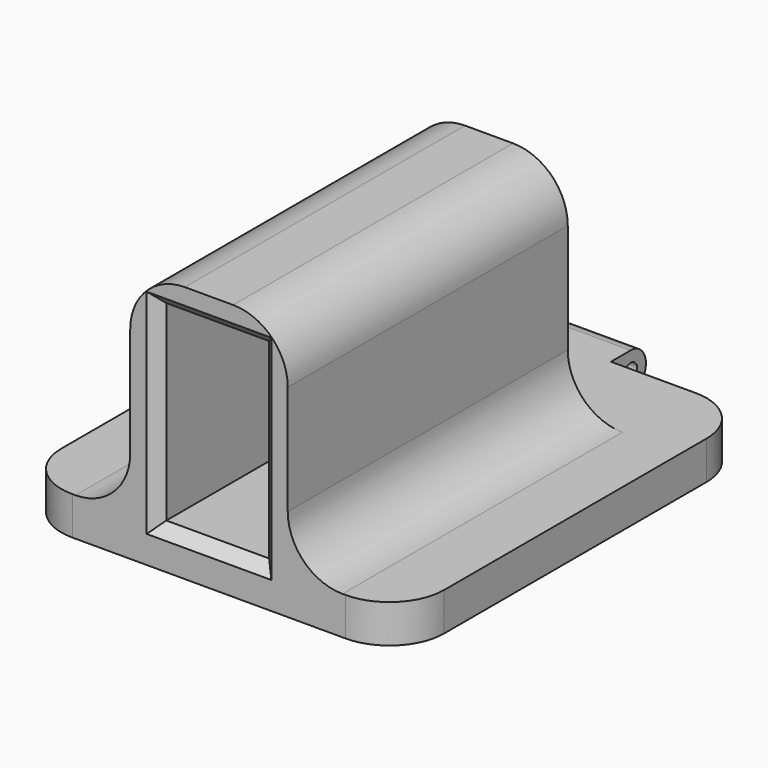
from build123d import *

# Parameters (mm, degrees)
F0_W     = 9.5
F0_H     = 4
F1_DEPTH = 3.5
F2_R     = 1.74999
F3_R     = 0.75
F4_DEPTH = 10
F5_W     = 2.5
F5_H     = 32
F6_DEPTH = 17.5
F7_W     = 14.4
F7_H     = 32
F8_DEPTH = 2.5
F9_R     = 5
F10_SIZE = 1


# Not quite as in the source:
# - a fillet or chamfer is up to 0.001 mm smaller than in the source, because OpenCascade refuses the exact size


with BuildPart() as f1:
    # F0 (on Top) → F1 (new body)
    with BuildSketch(Plane.XY):
        Polygon((0, 40), (0, 0), (35, 0), (35, 40), (22.25, 40), (12.75, 40), align=None)
        with Locations((17.5, 42)):
            Rectangle(F0_W, F0_H)
    extrude(amount=F1_DEPTH)

    # F2 (radius 1.75 in the source; OpenCascade refuses exactly that, so slightly less here)
    f2_edges = [f1.edges().sort_by_distance(p)[0] for p in [
        (17.5, 44, 3.5),
        (17.5, 44, 0),
    ]]
    fillet(f2_edges, radius=F2_R)

    # F3 (on face) → F4 (cut)
    with BuildSketch(Plane.YZ.offset(22.25)):
        with Locations((42.25, 1.75)):
            Circle(F3_R)
    extrude(amount=-F4_DEPTH, mode=Mode.SUBTRACT)

    # F5 (on face) → F6 (join)
    with BuildSketch(Plane.XY.offset(3.5)):
        with Locations((11.55, 16)):
            Rectangle(F5_W, F5_H)
        with Locations((23.45, 16)):
            Rectangle(F5_W, F5_H)
    extrude(amount=F6_DEPTH)

    # F7 (on face) → F8 (join)
    with BuildSketch(Plane.XY.offset(21)):
        with Locations((17.5, 16)):
            Rectangle(F7_W, F7_H)
    extrude(amount=F8_DEPTH)

    # F9
    f9_edges = [f1.edges().sort_by_distance(p)[0] for p in [
        (24.7, 16, 23.5),
        (10.3, 16, 23.5),
        (24.7, 16, 3.5),
        (10.3, 16, 3.5),
        (35, 40, 1.75),
        (0, 40, 1.75),
        (0, 0, 1.75),
        (35, 0, 1.75),
    ]]
    fillet(f9_edges, radius=F9_R)

    # F10
    f10_edges = [f1.edges().sort_by_distance(p)[0] for p in [
        (12.8, 0, 12.25),
        (17.5, 0, 3.5),
        (22.2, 0, 12.25),
        (17.5, 0, 21),
    ]]
    chamfer(f10_edges, length=F10_SIZE)


solid = f1.part
